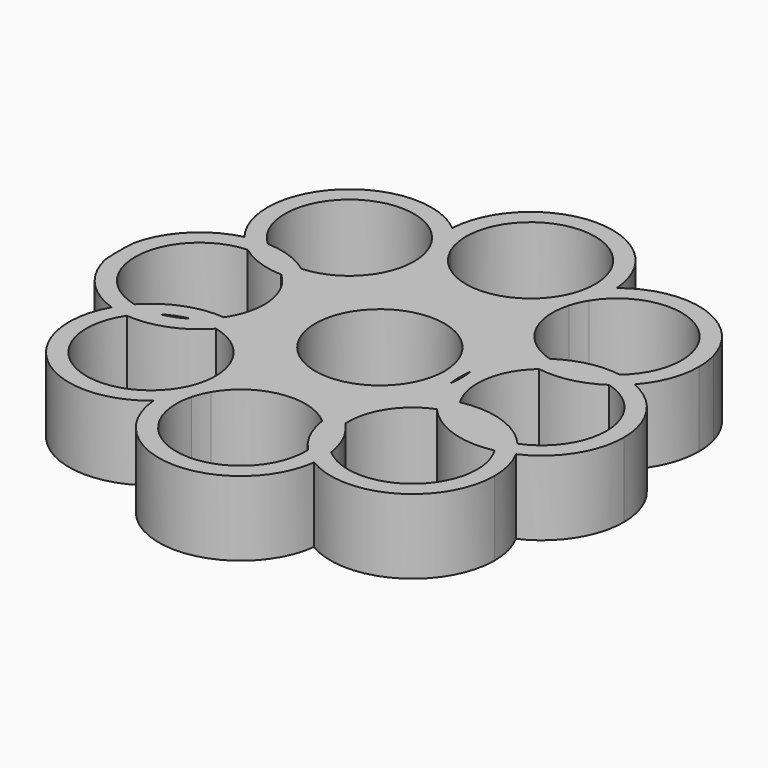
from build123d import *

# Parameters (mm, degrees)
F0_R     = 10.9982
F1_DEPTH = 12.7


with BuildPart() as f1:
    # F0 (on Top) → F1 (new body)
    with BuildSketch(Plane.XY):
        with BuildLine():
            ThreePointArc((36.6595053904, 22.1415615255), (36.5332921925, 24.0151855477), (36.1569331676, 25.8549547266))
            ThreePointArc((36.1569331676, 25.8549547266), (31.8126817374, 31.044416256), (26.7309490751, 35.514206475))
            ThreePointArc((26.7309490751, 35.514206475), (20.0275986163, 35.8556109759), (13.9387298404, 33.0312276028))
            ThreePointArc((13.9387298404, 33.0312276028), (13.9621802716, 32.5643943457), (13.97, 32.0970378816))
            ThreePointArc((13.97, 32.0970378816), (13.809120306, 29.9830141416), (13.3301866323, 27.9176809516))
            ThreePointArc((13.3301866323, 27.9176809516), (25.6915666552, 32.7221111995), (33.6877053904, 22.1415615255))
            ThreePointArc((33.6877053904, 22.1415615255), (32.6807162633, 17.5441591575), (29.8441476203, 13.7886280407))
            ThreePointArc((29.8441476203, 13.7886280407), (31.5063251421, 13.4128387201), (33.1103805724, 12.8374624052))
            ThreePointArc((33.1103805724, 12.8374624052), (35.7421014213, 17.1625418576), (36.6595053904, 22.1415615255))
        make_face()
        with BuildLine():
            ThreePointArc((26.7309490751, 35.514206475), (31.8126817374, 31.044416256), (36.1569331676, 25.8549547266))
            ThreePointArc((36.1569331676, 25.8549547266), (32.6877767936, 31.8983780631), (26.7309490751, 35.514206475))
        make_face()
        with BuildLine():
            ThreePointArc((-35.0731566807, -13.2683694138), (-36.7917944171, -21.5711650181), (-33.3923149137, -29.3386401304))
            ThreePointArc((-33.3923149137, -29.3386401304), (-23.9570048726, -34.0476963086), (-13.9180516707, -30.8197396373))
            ThreePointArc((-13.9180516707, -30.8197396373), (-13.8996752079, -28.2161297549), (-13.3984786946, -25.661149487))
            ThreePointArc((-13.3984786946, -25.661149487), (-28.776093154, -29.4132769471), (-31.9773540352, -13.9116184645))
            ThreePointArc((-31.9773540352, -13.9116184645), (-33.5435128628, -13.6778629095), (-35.0731566807, -13.2683694138))
        make_face()
        with BuildLine():
            ThreePointArc((-44.3500050785, 2.9798573019), (-44.45, 0), (-44.3500050785, -2.9798573019))
            ThreePointArc((-44.3500050785, -2.9798573019), (-41.0767090039, -9.3550091876), (-35.0731566807, -13.2683694138))
            ThreePointArc((-35.0731566807, -13.2683694138), (-34.2197857507, -11.9344829162), (-33.2209432758, -10.7057401266))
            ThreePointArc((-33.2209432758, -10.7057401266), (-41.6568779936, 0.9697265091), (-31.3012430481, 10.9818362069))
            ThreePointArc((-31.3012430481, 10.9818362069), (-32.7092505873, 12.1971076688), (-33.9433392044, 13.5886518621))
            ThreePointArc((-33.9433392044, 13.5886518621), (-40.6743431807, 9.7828190024), (-44.3500050785, 2.9798573019))
        make_face()
        with BuildLine():
            ThreePointArc((-33.2209432758, -10.7057401266), (-34.2197857507, -11.9344829162), (-35.0731566807, -13.2683694138))
            ThreePointArc((-35.0731566807, -13.2683694138), (-33.5435128628, -13.6778629095), (-31.9773540352, -13.9116184645))
            ThreePointArc((-31.9773540352, -13.9116184645), (-30.5399313145, -12.2087541474), (-28.7887583748, -10.8305943977))
            ThreePointArc((-28.7887583748, -10.8305943977), (-31.0112079738, -10.9938388171), (-33.2209432758, -10.7057401266))
        make_face()
        with BuildLine():
            ThreePointArc((-13.3984786946, -25.661149487), (-13.8996752079, -28.2161297549), (-13.9180516707, -30.8197396373))
            ThreePointArc((-13.9180516707, -30.8197396373), (-12.0881248548, -28.9675814469), (-10.6336762496, -26.8080209895))
            ThreePointArc((-10.6336762496, -26.8080209895), (-10.15886339, -25.4020923525), (-9.4991085531, -24.0728797514))
            ThreePointArc((-9.4991085531, -24.0728797514), (-9.0712058092, -22.1159428971), (-8.9275872476, -20.1179247995))
            ThreePointArc((-8.9275872476, -20.1179247995), (-8.9405803722, -19.5155469447), (-8.9795355769, -18.9142896011))
            ThreePointArc((-8.9795355769, -18.9142896011), (-10.8094623929, -20.7664477915), (-12.2639109981, -22.9260082489))
            ThreePointArc((-12.2639109981, -22.9260082489), (-12.7387238577, -24.3319368858), (-13.3984786946, -25.661149487))
        make_face()
        with BuildLine():
            ThreePointArc((-10.6336762496, -26.8080209895), (-12.0881248548, -28.9675814469), (-13.9180516707, -30.8197396373))
            ThreePointArc((-13.9180516707, -30.8197396373), (-0.2611307533, -43.5836636648), (13.8633362869, -31.3391270727))
            ThreePointArc((13.8633362869, -31.3391270727), (12.3461913769, -30.279208289), (10.9824672855, -29.0280435884))
            ThreePointArc((10.9824672855, -29.0280435884), (10.9942661178, -29.321968806), (10.9982, -29.6161044389))
            ThreePointArc((10.9982, -29.6161044389), (-1.415822219, -40.5227927852), (-10.6336762496, -26.8080209895))
        make_face()
        with BuildLine():
            ThreePointArc((13.9387298404, 33.0312276028), (12.059390514, 39.1491298005), (7.6490093808, 43.7869290484))
            ThreePointArc((7.6490093808, 43.7869290484), (0, 44.45), (-7.6490093808, 43.7869290484))
            ThreePointArc((-7.6490093808, 43.7869290484), (-12.1002142351, 39.0788510748), (-13.9486559845, 32.8689810311))
            ThreePointArc((-13.9486559845, 32.8689810311), (-11.7159971411, 30.5161028675), (-10.0861193168, 27.7117670386))
            ThreePointArc((-10.0861193168, 27.7117670386), (-2.2395586362, 42.8648036831), (10.9982, 32.0970378816))
            ThreePointArc((10.9982, 32.0970378816), (10.8951364792, 30.594904619), (10.587877522, 29.1209241709))
            ThreePointArc((10.587877522, 29.1209241709), (12.0815696669, 31.2318090297), (13.9387298404, 33.0312276028))
        make_face()
        with BuildLine():
            ThreePointArc((-7.6490093808, 43.7869290484), (0, 44.45), (7.6490093808, 43.7869290484))
            ThreePointArc((7.6490093808, 43.7869290484), (0, 46.0670378816), (-7.6490093808, 43.7869290484))
        make_face()
        with BuildLine():
            ThreePointArc((13.97, 32.0970378816), (13.9621802716, 32.5643943457), (13.9387298404, 33.0312276028))
            ThreePointArc((13.9387298404, 33.0312276028), (12.0815696669, 31.2318090297), (10.587877522, 29.1209241709))
            ThreePointArc((10.587877522, 29.1209241709), (10.0713786475, 27.678018151), (9.3593187581, 26.3209184555))
            ThreePointArc((9.3593187581, 26.3209184555), (8.8173915919, 23.7924275898), (8.7507755499, 21.2073718043))
            ThreePointArc((8.7507755499, 21.2073718043), (10.6079357234, 23.0067903774), (12.1016278684, 25.1176752363))
            ThreePointArc((12.1016278684, 25.1176752363), (12.6181267429, 26.5605812561), (13.3301866323, 27.9176809516))
            ThreePointArc((13.3301866323, 27.9176809516), (13.809120306, 29.9830141416), (13.97, 32.0970378816))
        make_face()
        with BuildLine():
            ThreePointArc((30.5525684391, 10.5945645354), (31.9000019579, 11.6378644155), (33.1103805724, 12.8374624052))
            ThreePointArc((33.1103805724, 12.8374624052), (31.5063251421, 13.4128387201), (29.8441476203, 13.7886280407))
            ThreePointArc((29.8441476203, 13.7886280407), (25.0709576069, 11.4042858664), (19.737284947, 11.5469969902))
            ThreePointArc((19.737284947, 11.5469969902), (18.3898514282, 10.5036971101), (17.1794728138, 9.3040991203))
            ThreePointArc((17.1794728138, 9.3040991203), (18.7835282441, 8.7287228054), (20.4457057658, 8.3529334848))
            ThreePointArc((20.4457057658, 8.3529334848), (25.2188957792, 10.7372756591), (30.5525684391, 10.5945645354))
        make_face()
        with BuildLine():
            ThreePointArc((41.5703479958, 0), (39.2651680779, 7.6871888524), (33.1103805724, 12.8374624052))
            ThreePointArc((33.1103805724, 12.8374624052), (31.9000019579, 11.6378644155), (30.5525684391, 10.5945645354))
            ThreePointArc((30.5525684391, 10.5945645354), (36.3590440779, 6.6517400866), (38.5985479958, 0))
            ThreePointArc((38.5985479958, 0), (36.6944361636, -6.1853022267), (31.6414161677, -10.2288890535))
            ThreePointArc((31.6414161677, -10.2288890535), (32.5730438121, -11.4291217528), (33.3688178772, -12.7234293815))
            ThreePointArc((33.3688178772, -12.7234293815), (39.3422904297, -7.5688630506), (41.5703479958, 0))
        make_face()
        with BuildLine():
            ThreePointArc((-28.7887583748, -10.8305943977), (-30.5399313145, -12.2087541474), (-31.9773540352, -13.9116184645))
            ThreePointArc((-31.9773540352, -13.9116184645), (-25.6492253052, -13.0244114798), (-20.3781564427, -9.4121846728))
            ThreePointArc((-20.3781564427, -9.4121846728), (-22.5878917447, -9.1240859824), (-24.8103413437, -9.2873304017))
            ThreePointArc((-24.8103413437, -9.2873304017), (-26.7239845749, -10.2537639468), (-28.7887583748, -10.8305943977))
        make_face()
        with BuildLine():
            ThreePointArc((-21.6217456833, -6.2063063349), (-27.9498744133, -7.0935133196), (-33.2209432758, -10.7057401266))
            ThreePointArc((-33.2209432758, -10.7057401266), (-31.0112079738, -10.9938388171), (-28.7887583748, -10.8305943977))
            ThreePointArc((-28.7887583748, -10.8305943977), (-26.8751151435, -9.8641608526), (-24.8103413437, -9.2873304017))
            ThreePointArc((-24.8103413437, -9.2873304017), (-23.059168404, -7.9091706521), (-21.6217456833, -6.2063063349))
        make_face()
        with BuildLine():
            ThreePointArc((10.9824672855, -29.0280435884), (12.3461913769, -30.279208289), (13.8633362869, -31.3391270727))
            ThreePointArc((13.8633362869, -31.3391270727), (13.9433085731, -30.4792649315), (13.97, -29.6161044389))
            ThreePointArc((13.97, -29.6161044389), (13.9350517356, -28.628565515), (13.8303818001, -27.6459675748))
            ThreePointArc((13.8303818001, -27.6459675748), (11.1933031436, -24.1840608478), (10.1054399692, -19.9703290409))
            ThreePointArc((10.1054399692, -19.9703290409), (8.7417158778, -18.7191643403), (7.2245709678, -17.6592455566))
            ThreePointArc((7.2245709678, -17.6592455566), (7.118463381, -19.5069191441), (7.2575254546, -21.3524050545))
            ThreePointArc((7.2575254546, -21.3524050545), (9.8946041111, -24.8143117814), (10.9824672855, -29.0280435884))
        make_face()
        with BuildLine():
            ThreePointArc((13.97, -29.6161044389), (13.9433085731, -30.4792649315), (13.8633362869, -31.3391270727))
            ThreePointArc((13.8633362869, -31.3391270727), (27.952076672, -31.5496047194), (35.0579072547, -19.3822681904))
            ThreePointArc((35.0579072547, -19.3822681904), (34.6290523576, -15.9474043937), (33.3688178772, -12.7234293815))
            ThreePointArc((33.3688178772, -12.7234293815), (31.9529542163, -13.2746268908), (30.4856051307, -13.6688035784))
            ThreePointArc((30.4856051307, -13.6688035784), (31.6784257505, -16.4155661106), (32.0861072547, -19.3822681904))
            ThreePointArc((32.0861072547, -19.3822681904), (25.6233612995, -29.4017522014), (13.8303818001, -27.6459675748))
            ThreePointArc((13.8303818001, -27.6459675748), (13.9350517356, -28.628565515), (13.97, -29.6161044389))
        make_face()
        with BuildLine():
            ThreePointArc((19.737284947, 11.5469969902), (25.0709576069, 11.4042858664), (29.8441476203, 13.7886280407))
            ThreePointArc((29.8441476203, 13.7886280407), (24.5754086907, 13.6385718534), (19.737284947, 11.5469969902))
        make_face()
        with BuildLine():
            ThreePointArc((20.4457057658, 8.3529334848), (25.7144446954, 8.5029896721), (30.5525684391, 10.5945645354))
            ThreePointArc((30.5525684391, 10.5945645354), (25.2188957792, 10.7372756591), (20.4457057658, 8.3529334848))
        make_face()
        with BuildLine():
            ThreePointArc((-26.6008057499, 35.6117906522), (-32.9402707471, 31.8526586896), (-36.4845167296, 25.390599422))
            ThreePointArc((-36.4845167296, 25.390599422), (-31.9539929528, 30.898945522), (-26.6008057499, 35.6117906522))
        make_face()
        with BuildLine():
            ThreePointArc((-26.6008057499, 35.6117906522), (-31.9539929528, 30.898945522), (-36.4845167296, 25.390599422))
            ThreePointArc((-36.4845167296, 25.390599422), (-36.554590589, 19.200956191), (-33.9433392044, 13.5886518621))
            ThreePointArc((-33.9433392044, 13.5886518621), (-32.1094541548, 13.8988704654), (-30.2506123073, 13.9627214053))
            ThreePointArc((-30.2506123073, 13.9627214053), (-29.326558574, 31.0650547274), (-12.8114679451, 26.5268324014))
            ThreePointArc((-12.8114679451, 26.5268324014), (-13.7507007273, 29.6314488023), (-13.9486559845, 32.8689810311))
            ThreePointArc((-13.9486559845, 32.8689810311), (-19.9378361185, 35.7944283766), (-26.6008057499, 35.6117906522))
        make_face()
        with BuildLine():
            ThreePointArc((-30.2506123073, 13.9627214053), (-32.1094541548, 13.8988704654), (-33.9433392044, 13.5886518621))
            ThreePointArc((-33.9433392044, 13.5886518621), (-32.7092505873, 12.1971076688), (-31.3012430481, 10.9818362069))
            ThreePointArc((-31.3012430481, 10.9818362069), (-27.0455661697, 10.3727749365), (-23.3484874112, 8.1788401202))
            ThreePointArc((-23.3484874112, 8.1788401202), (-21.4896455636, 8.2426910601), (-19.6557605141, 8.5529096634))
            ThreePointArc((-19.6557605141, 8.5529096634), (-20.8898491312, 9.9444538567), (-22.2978566704, 11.1597253186))
            ThreePointArc((-22.2978566704, 11.1597253186), (-26.5535335488, 11.768786589), (-30.2506123073, 13.9627214053))
        make_face()
        with BuildLine():
            ThreePointArc((-18.5259430378, -6.8495553856), (-19.3793139677, -8.1834418832), (-20.3781564427, -9.4121846728))
            ThreePointArc((-20.3781564427, -9.4121846728), (-14.2758238805, -13.289630746), (-11.8993872476, -20.1179247995))
            ThreePointArc((-11.8993872476, -20.1179247995), (-11.9908989013, -21.5337470185), (-12.2639109981, -22.9260082489))
            ThreePointArc((-12.2639109981, -22.9260082489), (-10.8094623929, -20.7664477915), (-8.9795355769, -18.9142896011))
            ThreePointArc((-8.9795355769, -18.9142896011), (-11.9423283838, -11.4494068623), (-18.5259430378, -6.8495553856))
        make_face()
        with BuildLine():
            ThreePointArc((-24.8103413437, -9.2873304017), (-22.5878917447, -9.1240859824), (-20.3781564427, -9.4121846728))
            ThreePointArc((-20.3781564427, -9.4121846728), (-19.3793139677, -8.1834418832), (-18.5259430378, -6.8495553856))
            ThreePointArc((-18.5259430378, -6.8495553856), (-20.0555868557, -6.4400618899), (-21.6217456833, -6.2063063349))
            ThreePointArc((-21.6217456833, -6.2063063349), (-23.059168404, -7.9091706521), (-24.8103413437, -9.2873304017))
        make_face()
        with BuildLine():
            ThreePointArc((-23.3484874112, 8.1788401202), (-27.0455661697, 10.3727749365), (-31.3012430481, 10.9818362069))
            ThreePointArc((-31.3012430481, 10.9818362069), (-27.5413989466, 8.9659813522), (-23.3484874112, 8.1788401202))
        make_face()
        with BuildLine():
            ThreePointArc((-19.7033124708, 0), (-20.1938606322, -3.248023411), (-21.6217456833, -6.2063063349))
            ThreePointArc((-21.6217456833, -6.2063063349), (-20.0555868557, -6.4400618899), (-18.5259430378, -6.8495553856))
            ThreePointArc((-18.5259430378, -6.8495553856), (-17.187564029, -3.5403527381), (-16.7315124708, 0))
            ThreePointArc((-16.7315124708, 0), (-17.4827747316, 4.5194991517), (-19.6557605141, 8.5529096634))
            ThreePointArc((-19.6557605141, 8.5529096634), (-21.4896455636, 8.2426910601), (-23.3484874112, 8.1788401202))
            ThreePointArc((-23.3484874112, 8.1788401202), (-20.655855612, 4.4771845522), (-19.7033124708, 0))
        make_face()
        with BuildLine():
            ThreePointArc((-8.9275872476, -20.1179247995), (-9.0712058092, -22.1159428971), (-9.4991085531, -24.0728797514))
            ThreePointArc((-9.4991085531, -24.0728797514), (-1.7625037137, -18.760046964), (7.2575254546, -21.3524050545))
            ThreePointArc((7.2575254546, -21.3524050545), (7.118463381, -19.5069191441), (7.2245709678, -17.6592455566))
            ThreePointArc((7.2245709678, -17.6592455566), (-1.0787766605, -15.6878187972), (-8.9795355769, -18.9142896011))
            ThreePointArc((-8.9795355769, -18.9142896011), (-8.9405803722, -19.5155469447), (-8.9275872476, -20.1179247995))
        make_face()
        with BuildLine():
            ThreePointArc((7.2575254546, -21.3524050545), (8.5197034185, -25.4815429285), (10.9824672855, -29.0280435884))
            ThreePointArc((10.9824672855, -29.0280435884), (9.8946041111, -24.8143117814), (7.2575254546, -21.3524050545))
        make_face()
        with BuildLine():
            ThreePointArc((-10.0861193168, 27.7117670386), (-11.7159971411, 30.5161028675), (-13.9486559845, 32.8689810311))
            ThreePointArc((-13.9486559845, 32.8689810311), (-13.7507007273, 29.6314488023), (-12.8114679451, 26.5268324014))
            ThreePointArc((-12.8114679451, 26.5268324014), (-11.1815901173, 23.7224965539), (-8.9489312631, 21.3696183761))
            ThreePointArc((-8.9489312631, 21.3696183761), (-8.932924271, 21.75544244), (-8.9275872476, 22.1415615255))
            ThreePointArc((-8.9275872476, 22.1415615255), (-9.2202865821, 24.9862665196), (-10.0861193168, 27.7117670386))
        make_face()
        with BuildLine():
            ThreePointArc((8.7507755499, 21.2073718043), (8.8173915919, 23.7924275898), (9.3593187581, 26.3209184555))
            ThreePointArc((9.3593187581, 26.3209184555), (-0.7846494175, 21.1268633829), (-10.0861193168, 27.7117670386))
            ThreePointArc((-10.0861193168, 27.7117670386), (-9.2202865821, 24.9862665196), (-8.9275872476, 22.1415615255))
            ThreePointArc((-8.9275872476, 22.1415615255), (-8.932924271, 21.75544244), (-8.9489312631, 21.3696183761))
            ThreePointArc((-8.9489312631, 21.3696183761), (-6.6028466768, 19.7859324981), (-3.9856875286, 18.707669154))
            ThreePointArc((-3.9856875286, 18.707669154), (2.6904728762, 18.3885640168), (8.7507755499, 21.2073718043))
        make_face()
        with BuildLine():
            ThreePointArc((30.4856051307, -13.6688035784), (31.9529542163, -13.2746268908), (33.3688178772, -12.7234293815))
            ThreePointArc((33.3688178772, -12.7234293815), (32.5730438121, -11.4291217528), (31.6414161677, -10.2288890535))
            ThreePointArc((31.6414161677, -10.2288890535), (29.9449474712, -10.7453830336), (28.1875230343, -10.9825146808))
            ThreePointArc((28.1875230343, -10.9825146808), (29.4452020606, -12.2327208784), (30.4856051307, -13.6688035784))
        make_face()
        with BuildLine():
            ThreePointArc((17.1794728138, 9.3040991203), (18.3898514282, 10.5036971101), (19.737284947, 11.5469969902))
            ThreePointArc((19.737284947, 11.5469969902), (13.1043924415, 16.7484165249), (12.1016278684, 25.1176752363))
            ThreePointArc((12.1016278684, 25.1176752363), (10.6079357234, 23.0067903774), (8.7507755499, 21.2073718043))
            ThreePointArc((8.7507755499, 21.2073718043), (11.288384172, 14.0684372874), (17.1794728138, 9.3040991203))
        make_face()
        with BuildLine():
            ThreePointArc((18.2026501198, -5.713464612), (16.7393683162, 1.731913289), (20.4457057658, 8.3529334848))
            ThreePointArc((20.4457057658, 8.3529334848), (18.7835282441, 8.7287228054), (17.1794728138, 9.3040991203))
            ThreePointArc((17.1794728138, 9.3040991203), (14.9756604504, 5.9814851318), (13.8001739979, 2.1716578064))
            ThreePointArc((13.8001739979, 2.1716578064), (13.9274787875, 1.0891439872), (13.97, 0))
            ThreePointArc((13.97, 0), (13.9274787875, -1.0891439872), (13.8001739979, -2.1716578064))
            ThreePointArc((13.8001739979, -2.1716578064), (14.3682112794, -4.4801180698), (15.3194373733, -6.6588388088))
            ThreePointArc((15.3194373733, -6.6588388088), (16.7353010341, -6.1076412996), (18.2026501198, -5.713464612))
        make_face()
        with BuildLine():
            ThreePointArc((-22.2978566704, 11.1597253186), (-26.0577007719, 13.1755801734), (-30.2506123073, 13.9627214053))
            ThreePointArc((-30.2506123073, 13.9627214053), (-26.5535335488, 11.768786589), (-22.2978566704, 11.1597253186))
        make_face()
        with BuildLine():
            ThreePointArc((-16.7315124708, 0), (-17.187564029, -3.5403527381), (-18.5259430378, -6.8495553856))
            ThreePointArc((-18.5259430378, -6.8495553856), (-11.9423283838, -11.4494068623), (-8.9795355769, -18.9142896011))
            ThreePointArc((-8.9795355769, -18.9142896011), (-1.0787766605, -15.6878187972), (7.2245709678, -17.6592455566))
            ThreePointArc((7.2245709678, -17.6592455566), (9.8360544956, -11.1023702751), (15.3194373733, -6.6588388088))
            ThreePointArc((15.3194373733, -6.6588388088), (14.3682112794, -4.4801180698), (13.8001739979, -2.1716578064))
            ThreePointArc((13.8001739979, -2.1716578064), (-10.6183557945, -9.0780735964), (0, 13.97))
            ThreePointArc((0, 13.97), (-1.8737816141, 16.4389987108), (-3.9856875286, 18.707669154))
            ThreePointArc((-3.9856875286, 18.707669154), (-6.6028466768, 19.7859324981), (-8.9489312631, 21.3696183761))
            ThreePointArc((-8.9489312631, 21.3696183761), (-12.176338273, 13.1852385957), (-19.6557605141, 8.5529096634))
            ThreePointArc((-19.6557605141, 8.5529096634), (-17.4827747316, 4.5194991517), (-16.7315124708, 0))
        make_face()
        with BuildLine():
            ThreePointArc((10.1054399692, -19.9703290409), (11.1933031436, -24.1840608478), (13.8303818001, -27.6459675748))
            ThreePointArc((13.8303818001, -27.6459675748), (12.5682038362, -23.5168297008), (10.1054399692, -19.9703290409))
        make_face()
        with BuildLine():
            ThreePointArc((-8.9489312631, 21.3696183761), (-11.1815901173, 23.7224965539), (-12.8114679451, 26.5268324014))
            ThreePointArc((-12.8114679451, 26.5268324014), (-12.1298214498, 24.3811201792), (-11.8993872476, 22.1415615255))
            ThreePointArc((-11.8993872476, 22.1415615255), (-14.9114630289, 14.5796686935), (-22.2978566704, 11.1597253186))
            ThreePointArc((-22.2978566704, 11.1597253186), (-20.8898491312, 9.9444538567), (-19.6557605141, 8.5529096634))
            ThreePointArc((-19.6557605141, 8.5529096634), (-12.176338273, 13.1852385957), (-8.9489312631, 21.3696183761))
        make_face()
        with BuildLine():
            ThreePointArc((17.1794728138, 9.3040991203), (11.288384172, 14.0684372874), (8.7507755499, 21.2073718043))
            ThreePointArc((8.7507755499, 21.2073718043), (2.6904728762, 18.3885640168), (-3.9856875286, 18.707669154))
            ThreePointArc((-3.9856875286, 18.707669154), (-1.8737816141, 16.4389987108), (0, 13.97))
            ThreePointArc((0, 13.97), (9.0780735964, 10.6183557945), (13.8001739979, 2.1716578064))
            ThreePointArc((13.8001739979, 2.1716578064), (14.9756604504, 5.9814851318), (17.1794728138, 9.3040991203))
        make_face()
        with BuildLine():
            ThreePointArc((28.1875230343, -10.9825146808), (29.9449474712, -10.7453830336), (31.6414161677, -10.2288890535))
            ThreePointArc((31.6414161677, -10.2288890535), (25.5373775383, -6.1397943205), (18.2026501198, -5.713464612))
            ThreePointArc((18.2026501198, -5.713464612), (19.2430531898, -7.149547312), (20.5007322161, -8.3997535096))
            ThreePointArc((20.5007322161, -8.3997535096), (24.5908538598, -8.956829671), (28.1875230343, -10.9825146808))
        make_face()
        with BuildLine():
            ThreePointArc((17.0468390827, -9.1533791368), (23.1508777121, -13.2424738699), (30.4856051307, -13.6688035784))
            ThreePointArc((30.4856051307, -13.6688035784), (29.4452020606, -12.2327208784), (28.1875230343, -10.9825146808))
            ThreePointArc((28.1875230343, -10.9825146808), (24.0974013906, -10.4254385194), (20.5007322161, -8.3997535096))
            ThreePointArc((20.5007322161, -8.3997535096), (18.7433077792, -8.6368851567), (17.0468390827, -9.1533791368))
        make_face()
        with BuildLine():
            ThreePointArc((20.5007322161, -8.3997535096), (19.2430531898, -7.149547312), (18.2026501198, -5.713464612))
            ThreePointArc((18.2026501198, -5.713464612), (16.7353010341, -6.1076412996), (15.3194373733, -6.6588388088))
            ThreePointArc((15.3194373733, -6.6588388088), (16.1152114383, -7.9531464375), (17.0468390827, -9.1533791368))
            ThreePointArc((17.0468390827, -9.1533791368), (18.7433077792, -8.6368851567), (20.5007322161, -8.3997535096))
        make_face()
        with BuildLine():
            ThreePointArc((15.3194373733, -6.6588388088), (9.8360544956, -11.1023702751), (7.2245709678, -17.6592455566))
            ThreePointArc((7.2245709678, -17.6592455566), (8.7417158778, -18.7191643403), (10.1054399692, -19.9703290409))
            ThreePointArc((10.1054399692, -19.9703290409), (11.8316523038, -13.442390454), (17.0468390827, -9.1533791368))
            ThreePointArc((17.0468390827, -9.1533791368), (16.1152114383, -7.9531464375), (15.3194373733, -6.6588388088))
        make_face()
        with BuildLine():
            ThreePointArc((20.5007322161, -8.3997535096), (24.0974013906, -10.4254385194), (28.1875230343, -10.9825146808))
            ThreePointArc((28.1875230343, -10.9825146808), (24.5908538598, -8.956829671), (20.5007322161, -8.3997535096))
        make_face()
        with BuildLine():
            ThreePointArc((13.8001739979, -2.1716578064), (13.6303479958, 0), (13.8001739979, 2.1716578064))
            ThreePointArc((13.8001739979, 2.1716578064), (9.0780735964, 10.6183557945), (0, 13.97))
            ThreePointArc((0, 13.97), (-10.6183557945, -9.0780735964), (13.8001739979, -2.1716578064))
        make_face()
        Circle(F0_R, mode=Mode.SUBTRACT)
    extrude(amount=F1_DEPTH)


solid = f1.part
